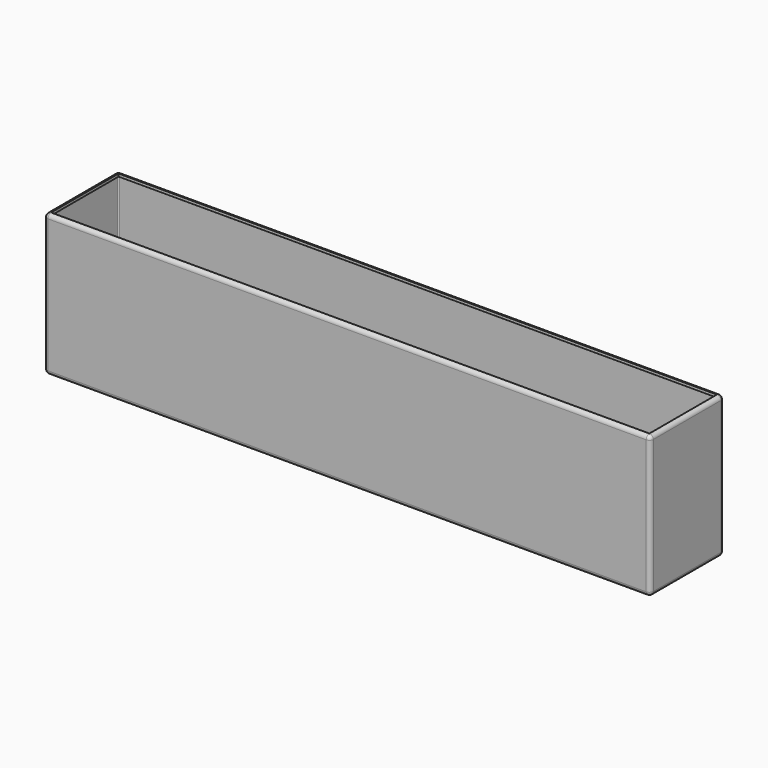
from build123d import *

# Parameters (mm, degrees)
F0_W     = 584.2
F0_H     = 136.525
F1_DEPTH = 88.9
F2_R     = 3.81
F3_T     = -2.54


# Not quite as in the source:
# - a shell that OpenCascade refuses in one call is made with other operations: the cavity is built on its own and cut out


with BuildPart() as f1:
    # F0 (on Front) → F1 (new body)
    with BuildSketch(Plane.XZ):
        Rectangle(F0_W, F0_H)
    extrude(amount=F1_DEPTH)

    # F2
    f2_edges = [f1.edges().sort_by_distance(p)[0] for p in [
        (-292.1, -44.45, 68.2625),
        (0, 0, 68.2625),
        (0, -88.9, 68.2625),
        (-292.1, -88.9, 0),
        (0, -88.9, -68.2625),
        (292.1, -88.9, 0),
        (292.1, -44.45, 68.2625),
        (-292.1, 0, 0),
        (-292.1, -44.45, -68.2625),
        (0, 0, -68.2625),
        (292.1, 0, 0),
        (292.1, -44.45, -68.2625),
    ]]
    fillet(f2_edges, radius=F2_R)

    # F3: a shell. OpenCascade refuses it in one call, so the cavity is built on its own and cut out:
    # the body offset inwards by the wall thickness, plus a prism from it out through each open face.
    f3_core = offset(f1.part, amount=F3_T, mode=Mode.PRIVATE)
    f3_exits = [f3_core.faces().sort_by_distance(p)[0] for p in [
        (0, -44.45, 65.7225),
    ]]
    add(f3_core, mode=Mode.SUBTRACT)
    extrude(f3_exits, amount=-F3_T, mode=Mode.SUBTRACT)


solid = f1.part
